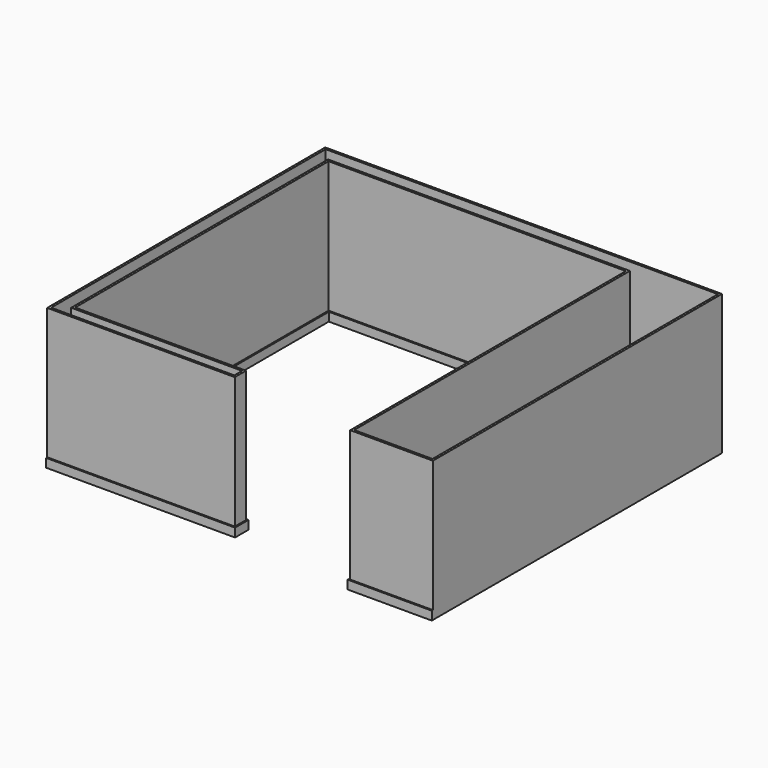
from build123d import *

# Parameters (mm, degrees)
F2_DEPTH = 0.6
F3_DEPTH = 1281.1125
F5_DEPTH = 79.375
F6_SCALE = 0.05
F8_DEPTH = 64.055625


with BuildPart() as f2:
    # F1 (on Top) → F2 (new body)
    with BuildSketch(Plane.XY):
        Polygon((-1358.9, -1320.8), (-1358.9, 1574.8), (1358.9, 1574.8), (1358.9, -1574.8), (2114.55, -1574.8), (2114.55, 1727.2), (-1511.3, 1727.2), (-1511.3, -1449.3875), (-1358.9, -1449.3875), (203.2, -1449.3875), (203.2, -1320.8), align=None)
    extrude(amount=F2_DEPTH)

    # F1 (on Top) → F3 (join)
    with BuildSketch(Plane.XY):
        Polygon((-1358.9, -1320.8), (-1358.9, 1574.8), (1358.9, 1574.8), (1358.9, -1574.8), (2114.55, -1574.8), (2114.55, 1727.2), (-1511.3, 1727.2), (-1511.3, -1449.3875), (-1358.9, -1449.3875), (203.2, -1449.3875), (203.2, -1320.8), align=None)
    extrude(amount=F3_DEPTH)

    # F4 (on Top) → F5 (join)
    with BuildSketch(Plane.XY):
        Polygon((203.2, -1320.8), (203.2, -1449.3875), (-1511.3, -1449.3875), (-1511.3, -1462.0875), (215.9, -1462.0875), (215.9, -1308.1), (-1346.2, -1308.1), (-1346.2, 1562.1), (1346.2, 1562.1), (1346.2, -1587.5), (2114.55, -1587.5), (2114.55, -1574.8), (1358.9, -1574.8), (1358.9, 1574.8), (-1358.9, 1574.8), (-1358.9, -1320.8), align=None)
    extrude(amount=F5_DEPTH)


with BuildPart() as f2_1:
    # F6: moved
    add(f2.part.scale(F6_SCALE))

    # F7 (on face) → F8 (cut, through all)
    with BuildSketch(Plane.XY.offset(64.055625)):
        Polygon((-68.945, -67.04), (-68.945, 79.74), (68.945, 79.74), (68.945, -77.74), (104.7275, -77.74), (104.7275, 85.36), (-74.565, 85.36), (-74.565, -71.469375), (9.16, -71.469375), (9.16, -67.04), align=None)
    extrude(amount=-F8_DEPTH, mode=Mode.SUBTRACT)


solid = f2_1.part
